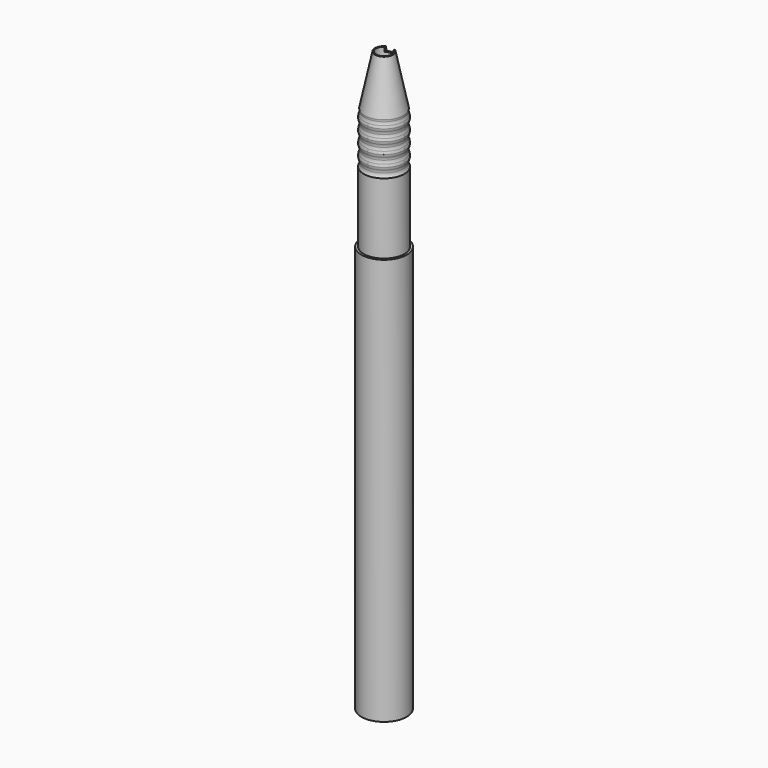
from build123d import *

# Parameters (mm, degrees)
F0_R      = 5
F1_DEPTH  = 90
F2_R      = 4.5
F3_DEPTH  = 26
F8_R      = 1.4999
F9_R      = 1.75
F10_DEPTH = 120
F12_DEPTH = 25


# Not quite as in the source:
# - a fillet or chamfer is up to 0.001 mm smaller than in the source, because OpenCascade refuses the exact size


with BuildPart() as f1:
    # F0 (on Top) → F1 (new body)
    with BuildSketch(Plane.XY):
        Circle(F0_R)
    extrude(amount=F1_DEPTH)

    # F2 (on face) → F3 (join)
    with BuildSketch(Plane.XY.offset(90)):
        Circle(F2_R)
    extrude(amount=F3_DEPTH)

    # F4 (on Right) → F5 (revolve)
    with BuildSketch(Plane.YZ):
        Polygon((-2, 128), (-4.5, 116), (0, 116), (0, 128), align=None)
    revolve(axis=Axis((0, 0, 122), (0, 0, -1)))

    # F6 (on Right) → F7 (revolve, cut)
    with BuildSketch(Plane.YZ):
        with BuildLine():
            ThreePointArc((-7.2247448714, 107.75), (-7.0844624167, 105.1265222001), (-4.5, 105.5986121811))
            Line((-4.5, 105.5986121811), (-4.5, 106.5))
            Line((-4.5, 106.5), (-6, 106.5))
            Line((-6, 106.5), (-6, 107.25))
            ThreePointArc((-6, 107.25), (-6.6614378278, 107.3798148254), (-7.2247448714, 107.75))
        make_face()
        with BuildLine():
            Line((-4.5, 106.5), (-4.5, 105.5986121811))
            ThreePointArc((-4.5, 105.5986121811), (-4.3136578046, 106.0322928267), (-4.25, 106.5))
            ThreePointArc((-4.25, 106.5), (-4.3866489029, 107.1779367504), (-4.7752551286, 107.75))
            ThreePointArc((-4.7752551286, 107.75), (-5.3385621722, 107.3798148254), (-6, 107.25))
            Line((-6, 107.25), (-6, 106.5))
            Line((-6, 106.5), (-4.5, 106.5))
        make_face()
        with BuildLine():
            ThreePointArc((-7.2247448714, 110.25), (-7.75, 109), (-7.2247448714, 107.75))
            ThreePointArc((-7.2247448714, 107.75), (-6.6614378278, 108.1201851746), (-6, 108.25))
            Line((-6, 108.25), (-6, 109))
            Line((-6, 109), (-6, 109.75))
            ThreePointArc((-6, 109.75), (-6.6614378278, 109.8798148254), (-7.2247448714, 110.25))
        make_face()
        with BuildLine():
            ThreePointArc((-6, 108.25), (-6.6614378278, 108.1201851746), (-7.2247448714, 107.75))
            ThreePointArc((-7.2247448714, 107.75), (-6.6614378278, 107.3798148254), (-6, 107.25))
            Line((-6, 107.25), (-6, 108.25))
        make_face()
        with BuildLine():
            Line((-6, 109), (-6, 108.25))
            ThreePointArc((-6, 108.25), (-5.3385621722, 108.1201851746), (-4.7752551286, 107.75))
            ThreePointArc((-4.7752551286, 107.75), (-4.3866489029, 108.3220632496), (-4.25, 109))
            ThreePointArc((-4.25, 109), (-4.3866489029, 109.6779367504), (-4.7752551286, 110.25))
            ThreePointArc((-4.7752551286, 110.25), (-5.3385621722, 109.8798148254), (-6, 109.75))
            Line((-6, 109.75), (-6, 109))
        make_face()
        with BuildLine():
            ThreePointArc((-4.7752551286, 107.75), (-5.3385621722, 108.1201851746), (-6, 108.25))
            Line((-6, 108.25), (-6, 107.25))
            ThreePointArc((-6, 107.25), (-5.3385621722, 107.3798148254), (-4.7752551286, 107.75))
        make_face()
        with BuildLine():
            ThreePointArc((-7.2247448714, 112.75), (-7.75, 111.5), (-7.2247448714, 110.25))
            ThreePointArc((-7.2247448714, 110.25), (-6.6614378278, 110.6201851746), (-6, 110.75))
            Line((-6, 110.75), (-6, 111.5))
            Line((-6, 111.5), (-6, 112.25))
            ThreePointArc((-6, 112.25), (-6.6614378278, 112.3798148254), (-7.2247448714, 112.75))
        make_face()
        with BuildLine():
            ThreePointArc((-6, 110.75), (-6.6614378278, 110.6201851746), (-7.2247448714, 110.25))
            ThreePointArc((-7.2247448714, 110.25), (-6.6614378278, 109.8798148254), (-6, 109.75))
            Line((-6, 109.75), (-6, 110.75))
        make_face()
        with BuildLine():
            Line((-6, 111.5), (-6, 110.75))
            ThreePointArc((-6, 110.75), (-5.3385621722, 110.6201851746), (-4.7752551286, 110.25))
            ThreePointArc((-4.7752551286, 110.25), (-4.3866489029, 110.8220632496), (-4.25, 111.5))
            ThreePointArc((-4.25, 111.5), (-4.3866489029, 112.1779367504), (-4.7752551286, 112.75))
            ThreePointArc((-4.7752551286, 112.75), (-5.3385621722, 112.3798148254), (-6, 112.25))
            Line((-6, 112.25), (-6, 111.5))
        make_face()
        with BuildLine():
            ThreePointArc((-4.7752551286, 110.25), (-5.3385621722, 110.6201851746), (-6, 110.75))
            Line((-6, 110.75), (-6, 109.75))
            ThreePointArc((-6, 109.75), (-5.3385621722, 109.8798148254), (-4.7752551286, 110.25))
        make_face()
        with BuildLine():
            ThreePointArc((-7.2247448714, 115.25), (-7.75, 114), (-7.2247448714, 112.75))
            ThreePointArc((-7.2247448714, 112.75), (-6.6614378278, 113.1201851746), (-6, 113.25))
            Line((-6, 113.25), (-6, 114))
            Line((-6, 114), (-6, 114.75))
            ThreePointArc((-6, 114.75), (-6.6614378278, 114.8798148254), (-7.2247448714, 115.25))
        make_face()
        with BuildLine():
            ThreePointArc((-6, 113.25), (-6.6614378278, 113.1201851746), (-7.2247448714, 112.75))
            ThreePointArc((-7.2247448714, 112.75), (-6.6614378278, 112.3798148254), (-6, 112.25))
            Line((-6, 112.25), (-6, 113.25))
        make_face()
        with BuildLine():
            Line((-6, 114), (-6, 113.25))
            ThreePointArc((-6, 113.25), (-5.3385621722, 113.1201851746), (-4.7752551286, 112.75))
            ThreePointArc((-4.7752551286, 112.75), (-4.3866489029, 113.3220632496), (-4.25, 114))
            ThreePointArc((-4.25, 114), (-4.3866489029, 114.6779367504), (-4.7752551286, 115.25))
            ThreePointArc((-4.7752551286, 115.25), (-5.3385621722, 114.8798148254), (-6, 114.75))
            Line((-6, 114.75), (-6, 114))
        make_face()
        with BuildLine():
            ThreePointArc((-4.7752551286, 112.75), (-5.3385621722, 113.1201851746), (-6, 113.25))
            Line((-6, 113.25), (-6, 112.25))
            ThreePointArc((-6, 112.25), (-5.3385621722, 112.3798148254), (-4.7752551286, 112.75))
        make_face()
        with BuildLine():
            ThreePointArc((-4.25, 116.5), (-6.6779367504, 118.1133510971), (-7.2247448714, 115.25))
            ThreePointArc((-7.2247448714, 115.25), (-6.6614378278, 115.6201851746), (-6, 115.75))
            ThreePointArc((-6, 115.75), (-5.3385621722, 115.6201851746), (-4.7752551286, 115.25))
            ThreePointArc((-4.7752551286, 115.25), (-4.3866489029, 115.8220632496), (-4.25, 116.5))
        make_face()
        with BuildLine():
            ThreePointArc((-6, 115.75), (-6.6614378278, 115.6201851746), (-7.2247448714, 115.25))
            ThreePointArc((-7.2247448714, 115.25), (-6.6614378278, 114.8798148254), (-6, 114.75))
            Line((-6, 114.75), (-6, 115.75))
        make_face()
        with BuildLine():
            ThreePointArc((-4.7752551286, 115.25), (-5.3385621722, 115.6201851746), (-6, 115.75))
            Line((-6, 115.75), (-6, 114.75))
            ThreePointArc((-6, 114.75), (-5.3385621722, 114.8798148254), (-4.7752551286, 115.25))
        make_face()
    revolve(axis=Axis((0, 0, 122), (0, 0, -1)), mode=Mode.SUBTRACT)

    # F8 (radius 1.5 in the source; OpenCascade refuses exactly that, so slightly less here)
    f8_edges = [f1.edges().sort_by_distance(p)[0] for p in [
        (-3.181981, 3.181981, 107.401388),
        (3.181981, -3.181981, 107.401388),
        (4.5, 0, 107.75),
        (3.181981, -3.181981, 108.098612),
        (-3.181981, 3.181981, 108.098612),
        (-3.181981, 3.181981, 109.901388),
        (3.181981, -3.181981, 109.901388),
        (4.5, 0, 110.25),
        (3.181981, -3.181981, 110.598612),
        (-3.181981, 3.181981, 110.598612),
        (-3.181981, 3.181981, 112.401388),
        (3.181981, -3.181981, 112.401388),
        (4.5, 0, 112.75),
        (3.181981, -3.181981, 113.098612),
        (-3.181981, 3.181981, 113.098612),
        (-3.181981, 3.181981, 114.901388),
        (3.181981, -3.181981, 114.901388),
        (4.5, 0, 115.25),
        (3.181981, -3.181981, 115.598612),
        (-3.181981, 3.181981, 115.598612),
    ]]
    fillet(f8_edges, radius=F8_R)

    # F9 (on face) → F10 (cut)
    with BuildSketch(Plane.XY.offset(128)):
        Circle(F9_R)
    extrude(amount=-F10_DEPTH, mode=Mode.SUBTRACT)

    # F11 (on Front) → F12 (cut)
    with BuildSketch(Plane.XZ):
        Polygon((-1, 127), (0, 127), (1, 127), (1, 128), (-1, 128), align=None)
    extrude(amount=-F12_DEPTH, mode=Mode.SUBTRACT)


solid = f1.part
